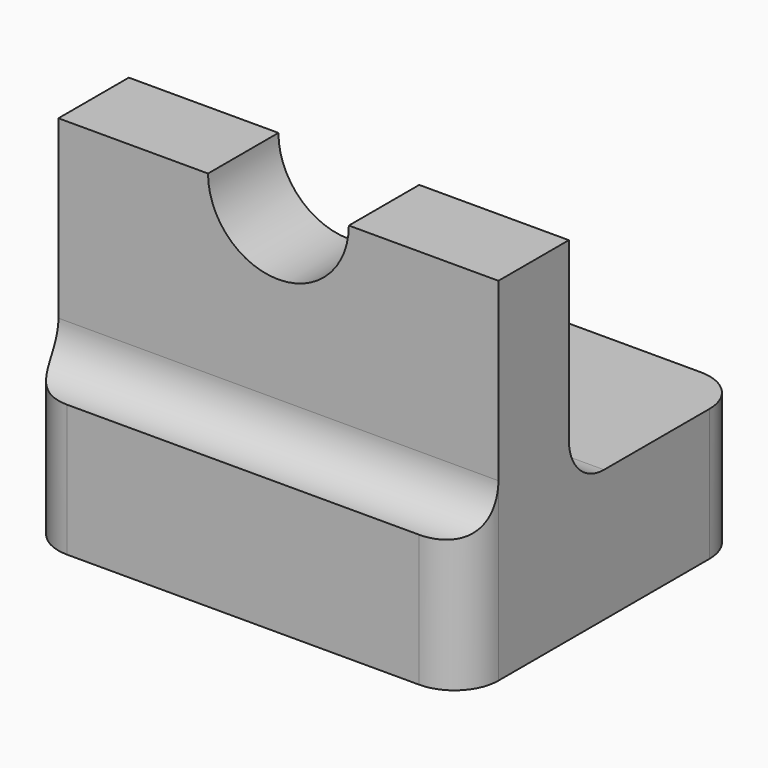
from build123d import *

# Parameters (mm, degrees)
F0_W        = 50
F0_H        = 40
F1_DEPTH    = 15
F2_W        = 50
F2_H        = 10
F3_DEPTH    = 25
F5_DEPTH    = 25
F7_T1_DEPTH = 50
F7_T3_DEPTH = 40


# Not quite as in the source:
# - a fillet or chamfer that OpenCascade refuses, or shapes differently, is made with other operations: its cross-section is extruded or revolved along the edge and cut away or added
# - a feature of the source that left no trace in its solid (it failed there, or was rolled back) is left out


with BuildPart() as f1:
    # F0 (on Top) → F1 (new body)
    with BuildSketch(Plane.XY):
        with Locations((29.4554777443, -26.2415218353)):
            Rectangle(F0_W, F0_H)
    extrude(amount=F1_DEPTH)

    # F2 (on face) → F3 (join)
    with BuildSketch(Plane.XY.offset(15)):
        with Locations((29.4554777443, -36.2415218353)):
            Rectangle(F2_W, F2_H)
    extrude(amount=F3_DEPTH)

    # F4 (on face) → F5 (cut)
    with BuildSketch(Plane(origin=(0, -31.2415218353, 0), x_dir=(-1, 0, 0), z_dir=(0, 1, 0))):
        with BuildLine():
            ThreePointArc((-37.4554777443, 40), (-29.4554777443, 32), (-21.4554777443, 40))
            Line((-21.4554777443, 40), (-37.4554777443, 40))
        make_face()
    extrude(amount=-F5_DEPTH, mode=Mode.SUBTRACT)

    # F7: fillet of radius 5 on 6 edges, made by hand

    # F7_s2 → F7_t1 (join)
    with BuildSketch(Plane.YZ.offset(4.4554777443)):
        with BuildLine():
            ThreePointArc((-46.2415218353, 15), (-42.7059879294, 16.4644660941), (-41.2415218353, 20))
            Line((-41.2415218353, 20), (-41.2415218353, 15))
            Line((-41.2415218353, 15), (-46.2415218353, 15))
        make_face()
        with BuildLine():
            ThreePointArc((-26.2415218353, 15), (-29.7770557413, 16.4644660941), (-31.2415218353, 20))
            Line((-31.2415218353, 20), (-31.2415218353, 15))
            Line((-31.2415218353, 15), (-26.2415218353, 15))
        make_face()
    extrude(amount=F7_T1_DEPTH)

    # F7_s4 → F7_t3 (cut)
    with BuildSketch(Plane.XY.offset(-12.5)):
        with BuildLine():
            ThreePointArc((9.4554777443, -46.2415218353), (5.9199438384, -44.7770557413), (4.4554777443, -41.2415218353))
            Line((4.4554777443, -41.2415218353), (4.4554777443, -46.2415218353))
            Line((4.4554777443, -46.2415218353), (9.4554777443, -46.2415218353))
        make_face()
        with BuildLine():
            ThreePointArc((49.4554777443, -46.2415218353), (52.9910116503, -44.7770557413), (54.4554777443, -41.2415218353))
            Line((54.4554777443, -41.2415218353), (54.4554777443, -46.2415218353))
            Line((54.4554777443, -46.2415218353), (49.4554777443, -46.2415218353))
        make_face()
        with BuildLine():
            ThreePointArc((4.4554777443, -11.2415218353), (5.9199438384, -7.7059879294), (9.4554777443, -6.2415218353))
            Line((9.4554777443, -6.2415218353), (4.4554777443, -6.2415218353))
            Line((4.4554777443, -6.2415218353), (4.4554777443, -11.2415218353))
        make_face()
        with BuildLine():
            ThreePointArc((54.4554777443, -11.2415218353), (52.9910116503, -7.7059879294), (49.4554777443, -6.2415218353))
            Line((49.4554777443, -6.2415218353), (54.4554777443, -6.2415218353))
            Line((54.4554777443, -6.2415218353), (54.4554777443, -11.2415218353))
        make_face()
    extrude(amount=F7_T3_DEPTH, mode=Mode.SUBTRACT)


solid = f1.part
